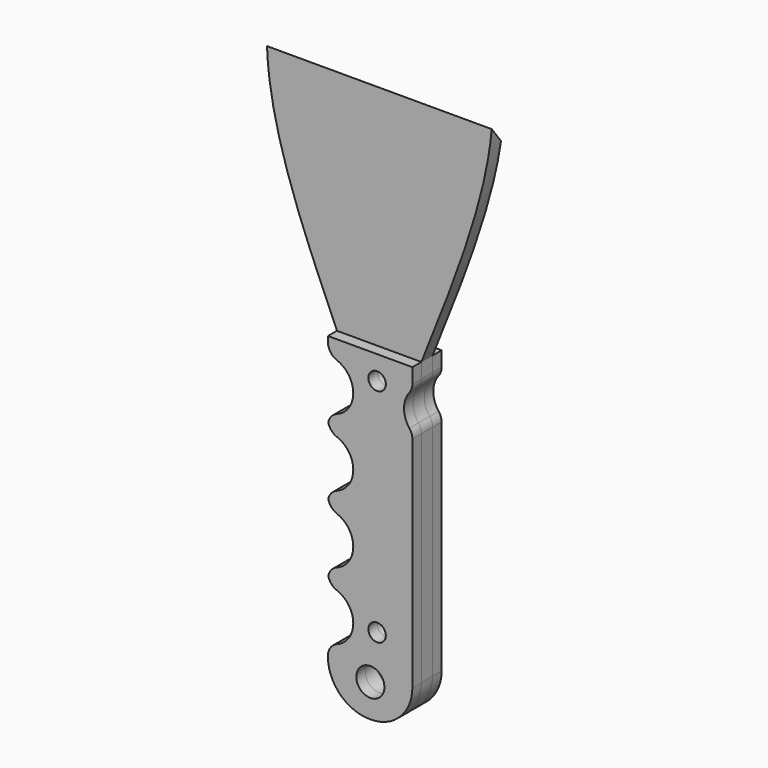
from build123d import *

# Parameters (mm, degrees)
F1_W          = 30
F1_H          = 85
F1_H_2        = 115
F2_DEPTH      = 5
F4_DEPTH      = 25
F5_T1_DEPTH   = 25.3834841531
F5_T3_DEPTH   = 14.7151745099
F6_R          = 14.7267027305
F8_DEPTH      = 4
F10_DEPTH     = 4
F11_R         = 3.1
F11_R_2       = 5
F12_DEPTH     = 25
F13_T1_DEPTH  = 131.4627937487
F14_TEXT_SIZE = 8.1223427882
F15_DEPTH     = 0.5


# Not quite as in the source:
# - a fillet or chamfer that OpenCascade refuses, or shapes differently, is made with other operations: its cross-section is extruded or revolved along the edge and cut away or added
# - Text() gives the source's letters only with a copy of the font that has no kerning and outlines rounded to 1/6400 em; it was checked with that copy


with BuildPart() as f2:
    # F1 (on face) → F2 (new body)
    with BuildSketch(Plane.XZ):
        with Locations((-2.4676704407, 106.1961215734)):
            Rectangle(F1_W, F1_H)
        with BuildLine():
            add(Edge.make_bspline(
                [(-17.4676704407, 63.6961215734), (-30.0253170876, 92.3866981237), (-42.5829637345, 121.077274674), (-42.3823421225, 148.6961215735)],
                knots=[0, 0, 0, 0, 0.5075570604, 0.5075570604, 0.5075570604, 0.5075570604], degree=3))
            Line((-17.4676704407, 63.6961215734), (-17.4676704407, 148.6961215734))
            Line((-17.4676704407, 148.6961215734), (-42.3823421225, 148.6961215734))
        make_face()
        with Locations((-2.4676704407, 6.1961215734)):
            Rectangle(F1_W, F1_H_2)
        with BuildLine():
            Line((12.5323295593, 148.6961215734), (12.5323295593, 63.6961215734))
            add(Edge.make_bspline(
                [(12.5323295593, 63.6961215734), (24.0723365112, 92.5131982023), (35.6123434632, 121.3302748311), (37.5323295593, 144.9015603046)],
                knots=[0, 0, 0, 0, 0.5466787046, 0.5466787046, 0.5466787046, 0.5466787046], degree=3))
            Line((37.5323295593, 144.9015603046), (37.5323295593, 148.6961215734))
            Line((37.5323295593, 148.6961215734), (12.5323295593, 148.6961215734))
        make_face()
    extrude(amount=F2_DEPTH)

    # F3 (on face) → F4 (cut)
    with BuildSketch(Plane.XZ.offset(5)):
        with BuildLine():
            ThreePointArc((-17.4676704407, 39.7464138567), (-11.10370941, 42.3824528261), (-8.4676704407, 48.7464138567))
            ThreePointArc((-8.4676704407, 48.7464138567), (-11.10370941, 55.1103748874), (-17.4676704407, 57.7464138567))
            Line((-17.4676704407, 57.7464138567), (-17.4676704407, 39.7464138567))
        make_face()
        with BuildLine():
            ThreePointArc((-8.4676704407, 24.7464138567), (-11.10370941, 31.1103748874), (-17.4676704407, 33.7464138567))
            Line((-17.4676704407, 33.7464138567), (-17.4676704407, 15.7464138567))
            ThreePointArc((-17.4676704407, 15.7464138567), (-11.10370941, 18.3824528261), (-8.4676704407, 24.7464138567))
        make_face()
        with BuildLine():
            ThreePointArc((-8.4676704407, 0.7464138567), (-11.10370941, 7.1103748874), (-17.4676704407, 9.7464138567))
            Line((-17.4676704407, 9.7464138567), (-17.4676704407, -8.2535861433))
            ThreePointArc((-17.4676704407, -8.2535861433), (-11.10370941, -5.6175471739), (-8.4676704407, 0.7464138567))
        make_face()
        with BuildLine():
            ThreePointArc((-8.4676704407, -23.2535861433), (-11.10370941, -16.8896251126), (-17.4676704407, -14.2535861433))
            Line((-17.4676704407, -14.2535861433), (-17.4676704407, -32.2535861433))
            ThreePointArc((-17.4676704407, -32.2535861433), (-11.10370941, -29.6175471739), (-8.4676704407, -23.2535861433))
        make_face()
        with BuildLine():
            Line((12.5323295593, 43.1544200206), (12.5323295593, 56.5277993059))
            ThreePointArc((12.5323295593, 56.5277993059), (9.5562968254, 49.8411096632), (12.5323295593, 43.1544200206))
        make_face()
    extrude(amount=-F4_DEPTH, mode=Mode.SUBTRACT)

    # F5: fillet of radius 5 on 10 edges, made by hand

    # F5_s2 → F5_t1 (cut)
    with BuildSketch(Plane.XZ.offset(-10.1917420766)):
        with BuildLine():
            ThreePointArc((-14.2533847264, -14.8471381807), (-16.5864427959, -13.0116228602), (-17.4676704407, -10.1768893126))
            Line((-17.4676704407, -10.1768893126), (-17.4676704407, -14.2535861433))
            ThreePointArc((-17.4676704407, -14.2535861433), (-15.8333558539, -14.4032180248), (-14.2533847264, -14.8471381807))
        make_face()
        with BuildLine():
            ThreePointArc((-17.4676704407, -12.3302829739), (-16.5864427959, -9.4955494263), (-14.2533847264, -7.6600341058))
            ThreePointArc((-14.2533847264, -7.6600341058), (-15.8333558539, -8.1039542617), (-17.4676704407, -8.2535861433))
            Line((-17.4676704407, -8.2535861433), (-17.4676704407, -12.3302829739))
        make_face()
        with BuildLine():
            ThreePointArc((-14.2533847264, 9.1528618193), (-16.5864427959, 10.9883771398), (-17.4676704407, 13.8231106874))
            Line((-17.4676704407, 13.8231106874), (-17.4676704407, 9.7464138567))
            ThreePointArc((-17.4676704407, 9.7464138567), (-15.8333558539, 9.5967819752), (-14.2533847264, 9.1528618193))
        make_face()
        with BuildLine():
            ThreePointArc((-17.4676704407, 11.6697170261), (-16.5864427959, 14.5044505737), (-14.2533847264, 16.3399658942))
            ThreePointArc((-14.2533847264, 16.3399658942), (-15.8333558539, 15.8960457383), (-17.4676704407, 15.7464138567))
            Line((-17.4676704407, 15.7464138567), (-17.4676704407, 11.6697170261))
        make_face()
        with BuildLine():
            ThreePointArc((-14.2533847264, 33.1528618193), (-16.5864427959, 34.9883771398), (-17.4676704407, 37.8231106874))
            Line((-17.4676704407, 37.8231106874), (-17.4676704407, 33.7464138567))
            ThreePointArc((-17.4676704407, 33.7464138567), (-15.8333558539, 33.5967819752), (-14.2533847264, 33.1528618193))
        make_face()
        with BuildLine():
            ThreePointArc((-14.2533847264, 40.3399658942), (-16.5864427959, 38.5044505737), (-17.4676704407, 35.6697170261))
            Line((-17.4676704407, 35.6697170261), (-17.4676704407, 39.7464138567))
            ThreePointArc((-17.4676704407, 39.7464138567), (-15.8333558539, 39.8960457383), (-14.2533847264, 40.3399658942))
        make_face()
        with BuildLine():
            ThreePointArc((-17.4676704407, 61.8231106874), (-16.5864427959, 58.9883771398), (-14.2533847264, 57.1528618193))
            ThreePointArc((-14.2533847264, 57.1528618193), (-15.8333558539, 57.5967819752), (-17.4676704407, 57.7464138567))
            Line((-17.4676704407, 57.7464138567), (-17.4676704407, 61.8231106874))
        make_face()
        with BuildLine():
            ThreePointArc((-17.4676704407, -36.3302829739), (-16.5864427959, -33.4955494263), (-14.2533847264, -31.6600341058))
            ThreePointArc((-14.2533847264, -31.6600341058), (-15.8333558539, -32.1039542617), (-17.4676704407, -32.2535861433))
            Line((-17.4676704407, -32.2535861433), (-17.4676704407, -36.3302829739))
        make_face()
    extrude(amount=F5_T1_DEPTH, mode=Mode.SUBTRACT)

    # F5_s4 → F5_t3 (cut)
    with BuildSketch(Plane.XZ.offset(-4.857587255)):
        with BuildLine():
            ThreePointArc((12.5323295593, 58.4708342079), (12.2591496232, 56.8407507487), (11.4694607258, 55.3887897277))
            ThreePointArc((11.4694607258, 55.3887897277), (11.9762035944, 55.9813354793), (12.5323295593, 56.5277993059))
            Line((12.5323295593, 56.5277993059), (12.5323295593, 58.4708342079))
        make_face()
        with BuildLine():
            ThreePointArc((11.4694607258, 44.2934295988), (12.2591496232, 42.8414685778), (12.5323295593, 41.2113851186))
            Line((12.5323295593, 41.2113851186), (12.5323295593, 43.1544200206))
            ThreePointArc((12.5323295593, 43.1544200206), (11.9762035944, 43.7008838472), (11.4694607258, 44.2934295988))
        make_face()
    extrude(amount=F5_T3_DEPTH, mode=Mode.SUBTRACT)

    # F6
    f6_edges = [f2.edges().sort_by_distance(p)[0] for p in [
        (12.53233, -2.5, -51.303878),
        (-17.46767, -2.5, -51.303878),
    ]]
    fillet(f6_edges, radius=F6_R)


with BuildPart() as f8:
    # F7 (on face) → F8 (new body)
    with BuildSketch(Plane.XZ.offset(5)):
        with BuildLine():
            Line((12.5323295593, 63.6961215734), (-17.4676704407, 63.6961215734))
            Line((-17.4676704407, 63.6961215734), (-17.4676704407, 61.8231106874))
            ThreePointArc((-17.4676704407, 61.8231106874), (-16.5864427959, 58.9883771398), (-14.2533847264, 57.1528618193))
            ThreePointArc((-14.2533847264, 57.1528618193), (-8.4676704407, 48.7464138567), (-14.2533847264, 40.3399658942))
            ThreePointArc((-14.2533847264, 40.3399658942), (-16.2551932804, 38.9338663392), (-17.3503668202, 36.7464138568))
            ThreePointArc((-17.3503668202, 36.7464138568), (-16.2551932804, 34.5589613743), (-14.2533847264, 33.1528618193))
            ThreePointArc((-14.2533847264, 33.1528618193), (-8.4676704407, 24.7464138567), (-14.2533847264, 16.3399658942))
            ThreePointArc((-14.2533847264, 16.3399658942), (-16.2551932804, 14.9338663392), (-17.3503668202, 12.7464138567))
            ThreePointArc((-17.3503668202, 12.7464138567), (-16.2551932804, 10.5589613743), (-14.2533847264, 9.1528618193))
            ThreePointArc((-14.2533847264, 9.1528618193), (-8.4676704407, 0.7464138567), (-14.2533847264, -7.6600341058))
            ThreePointArc((-14.2533847264, -7.6600341058), (-16.2551932804, -9.0661336608), (-17.3503668202, -11.2535861432))
            ThreePointArc((-17.3503668202, -11.2535861432), (-16.2551932804, -13.4410386257), (-14.2533847264, -14.8471381807))
            ThreePointArc((-14.2533847264, -14.8471381807), (-8.4676704407, -23.2535861433), (-14.2533847264, -31.6600341058))
            ThreePointArc((-14.2533847264, -31.6600341058), (-16.5864427959, -33.4955494263), (-17.4676704407, -36.3302829739))
            Line((-17.4676704407, -36.3302829739), (-17.4676704407, -36.5771756961))
            ThreePointArc((-17.4676704407, -36.5771756961), (-13.1543190754, -46.9905270613), (-2.7409677102, -51.3038784266))
            Line((-2.7409677102, -51.3038784266), (-2.1943731711, -51.3038784266))
            ThreePointArc((-2.1943731711, -51.3038784266), (8.2189781941, -46.9905270613), (12.5323295593, -36.5771756961))
            Line((12.5323295593, -36.5771756961), (12.5323295593, 41.2113851186))
            ThreePointArc((12.5323295593, 41.2113851186), (12.2591496232, 42.8414685778), (11.4694607258, 44.2934295988))
            ThreePointArc((11.4694607258, 44.2934295988), (9.5562968254, 49.8411096632), (11.4694607258, 55.3887897277))
            ThreePointArc((11.4694607258, 55.3887897277), (12.2591496232, 56.8407507487), (12.5323295593, 58.4708342079))
            Line((12.5323295593, 58.4708342079), (12.5323295593, 63.6961215734))
        make_face()
    extrude(amount=F8_DEPTH)


with BuildPart() as f10:
    # F9 (on face) → F10 (new body)
    with BuildSketch(Plane(origin=(0, 0, 0), x_dir=(-1, 0, 0), z_dir=(0, 1, 0))):
        with BuildLine():
            Line((17.4676704407, 63.6961215734), (-12.5323295593, 63.6961215734))
            Line((-12.5323295593, 63.6961215734), (-12.5323295593, 58.4708342079))
            ThreePointArc((-12.5323295593, 58.4708342079), (-12.2591496232, 56.8407507487), (-11.4694607258, 55.3887897277))
            ThreePointArc((-11.4694607258, 55.3887897277), (-9.5562968254, 49.8411096632), (-11.4694607258, 44.2934295988))
            ThreePointArc((-11.4694607258, 44.2934295988), (-12.2591496232, 42.8414685778), (-12.5323295593, 41.2113851186))
            Line((-12.5323295593, 41.2113851186), (-12.5323295593, -36.5771756961))
            ThreePointArc((-12.5323295593, -36.5771756961), (-8.2189781941, -46.9905270613), (2.1943731711, -51.3038784266))
            Line((2.1943731711, -51.3038784266), (2.7409677102, -51.3038784266))
            ThreePointArc((2.7409677102, -51.3038784266), (13.1543190754, -46.9905270613), (17.4676704407, -36.5771756961))
            Line((17.4676704407, -36.5771756961), (17.4676704407, -36.3302829739))
            ThreePointArc((17.4676704407, -36.3302829739), (16.5864427959, -33.4955494263), (14.2533847264, -31.6600341058))
            ThreePointArc((14.2533847264, -31.6600341058), (8.4676704407, -23.2535861433), (14.2533847264, -14.8471381807))
            ThreePointArc((14.2533847264, -14.8471381807), (16.2551932804, -13.4410386257), (17.3503668202, -11.2535861432))
            ThreePointArc((17.3503668202, -11.2535861432), (16.2551932804, -9.0661336608), (14.2533847264, -7.6600341058))
            ThreePointArc((14.2533847264, -7.6600341058), (8.4676704407, 0.7464138567), (14.2533847264, 9.1528618193))
            ThreePointArc((14.2533847264, 9.1528618193), (16.2551932804, 10.5589613743), (17.3503668202, 12.7464138567))
            ThreePointArc((17.3503668202, 12.7464138567), (16.2551932804, 14.9338663392), (14.2533847264, 16.3399658942))
            ThreePointArc((14.2533847264, 16.3399658942), (8.4676704407, 24.7464138567), (14.2533847264, 33.1528618193))
            ThreePointArc((14.2533847264, 33.1528618193), (16.2551932804, 34.5589613743), (17.3503668202, 36.7464138568))
            ThreePointArc((17.3503668202, 36.7464138568), (16.2551932804, 38.9338663392), (14.2533847264, 40.3399658942))
            ThreePointArc((14.2533847264, 40.3399658942), (8.4676704407, 48.7464138567), (14.2533847264, 57.1528618193))
            ThreePointArc((14.2533847264, 57.1528618193), (16.5864427959, 58.9883771398), (17.4676704407, 61.8231106874))
            Line((17.4676704407, 61.8231106874), (17.4676704407, 63.6961215734))
        make_face()
    extrude(amount=F10_DEPTH)


with BuildPart() as f12_tool:
    # F11 (on face) → F12 (new body)
    with BuildSketch(Plane(origin=(0, 4, 0), x_dir=(-1, 0, 0), z_dir=(0, 1, 0))):
        with Locations((0, 55.2614594619)):
            Circle(F11_R)
        with Locations((0, -23.3297403902)):
            Circle(F11_R)
        with Locations((2.3960061371, -39.6228432655)):
            Circle(F11_R_2)
    extrude(amount=-F12_DEPTH)


with BuildPart() as f2_1:
    add(f2.part)

    # F12: cut by f12_tool
    add(f12_tool.part, mode=Mode.SUBTRACT)

    # F13: chamfer of 10 x 8.3909963118 on 1 edges, made by hand

    # F13_s2 → F13_t1 (cut)
    with BuildSketch(Plane.YZ.offset(-68.1564031559)):
        Polygon((0, 138.6961215734), (-8.3909963118, 148.6961215734), (0, 148.6961215734), align=None)
    extrude(amount=F13_T1_DEPTH, mode=Mode.SUBTRACT)


with BuildPart() as f8_1:
    add(f8.part)

    # F12: cut by f12_tool
    add(f12_tool.part, mode=Mode.SUBTRACT)


with BuildPart() as f10_1:
    add(f10.part)

    # F12: cut by f12_tool
    add(f12_tool.part, mode=Mode.SUBTRACT)

    # F14 (on face) → F15 (cut)
    with BuildSketch(Plane(origin=(0, 4, 0), x_dir=(-1, 0, 0), z_dir=(0, 1, 0))):
        with Locations((-10, 9.4245794809)):
            Text('Haro', F14_TEXT_SIZE, font='Open Sans', font_style=FontStyle.BOLD, text_align=(TextAlign.LEFT, TextAlign.BOTTOM))
    extrude(amount=-F15_DEPTH, mode=Mode.SUBTRACT)


solid = Compound([f2_1.part, f8_1.part, f10_1.part])
